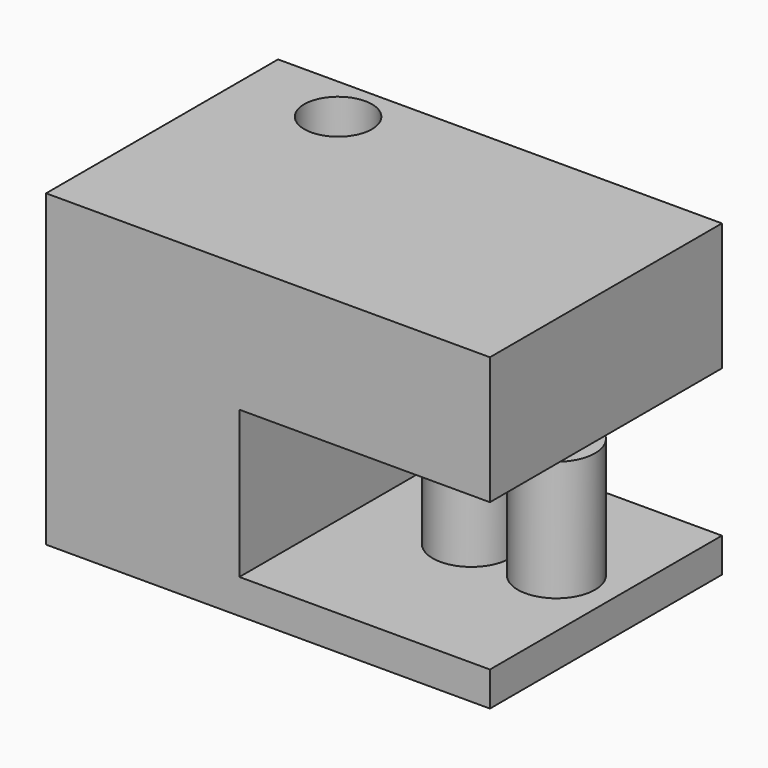
from build123d import *

# Parameters (mm, degrees)
F0_W           = 50
F0_H           = 75
F1_DEPTH       = 80
F2_D           = 3.3
F2_DEPTH       = 50
F2_CSINK_D     = 8.96
F2_CSINK_ANGLE = 90
F2_TIP         = 0.9914200214
F3_D           = 8.8
F3_DEPTH       = 20
F3_TIP         = 2.6437867237
F4_D           = 17.5
F5_W           = 75
F5_H           = 33.0074074864
F5_H_2         = 8.9014992118
F6_DEPTH       = 64.8
F8_R           = 10
F9_DEPTH       = 14.0455466509
F9_DEPTH_BACK  = 17.0455466509


with BuildPart() as f1:
    # F0 (on Top) → F1 (new body)
    with BuildSketch(Plane.XY):
        with Locations((-25, 0)):
            Rectangle(F0_W, F0_H)
    extrude(amount=F1_DEPTH)

    # F2
    with Locations(Plane(origin=(0, 0, 0), x_dir=(1, 0, 0), z_dir=(0, 0, -1))):
        with Locations((-34.0844392776, 22.1183039248), (40, 24.5), (40, -25.5), (-24.8667737842, -25.5)):
            CounterSinkHole(F2_D / 2, F2_CSINK_D / 2, depth=F2_DEPTH, counter_sink_angle=F2_CSINK_ANGLE)
            with Locations((0, 0, -(F2_DEPTH + F2_TIP / 2))):  # 118° drill point
                Cone(0, F2_D / 2, F2_TIP, mode=Mode.SUBTRACT)

    # F3
    with Locations(Plane(origin=(0, 0, 0), x_dir=(1, 0, 0), z_dir=(0, 0, -1))):
        with Locations((-34.0844392776, 22.1183039248)):
            Hole(F3_D / 2, depth=F3_DEPTH)
            with Locations((0, 0, -(F3_DEPTH + F3_TIP / 2))):  # 118° drill point
                Cone(0, F3_D / 2, F3_TIP, mode=Mode.SUBTRACT)

    # F4 (through all)
    with Locations(Plane(origin=(0, 0, 0), x_dir=(1, 0, 0), z_dir=(0, 0, -1))):
        with Locations((-24.8667737842, -25.5)):
            Hole(F4_D / 2)

    # F5 (on face) → F6 (join)
    with BuildSketch(Plane.YZ):
        with Locations((0, 63.4962962568)):
            Rectangle(F5_W, F5_H)
        with Locations((0, 4.4507496059)):
            Rectangle(F5_W, F5_H_2)
    extrude(amount=F6_DEPTH)


with BuildPart() as f9:
    # F8 (on mid) → F9 (new body, two sides)
    with BuildSketch(Plane.XY.offset(27.9470458627)) as f9_sk:
        with Locations((30, 0)):
            Circle(F8_R)
    extrude(amount=F9_DEPTH)
    extrude(f9_sk.sketch, amount=-F9_DEPTH_BACK)


with BuildPart() as f10_1:
    # F10: copy of F9
    add(f9.part.moved(Location((22, 0, 0))))


solid = Compound([f1.part, f9.part, f10_1.part])
